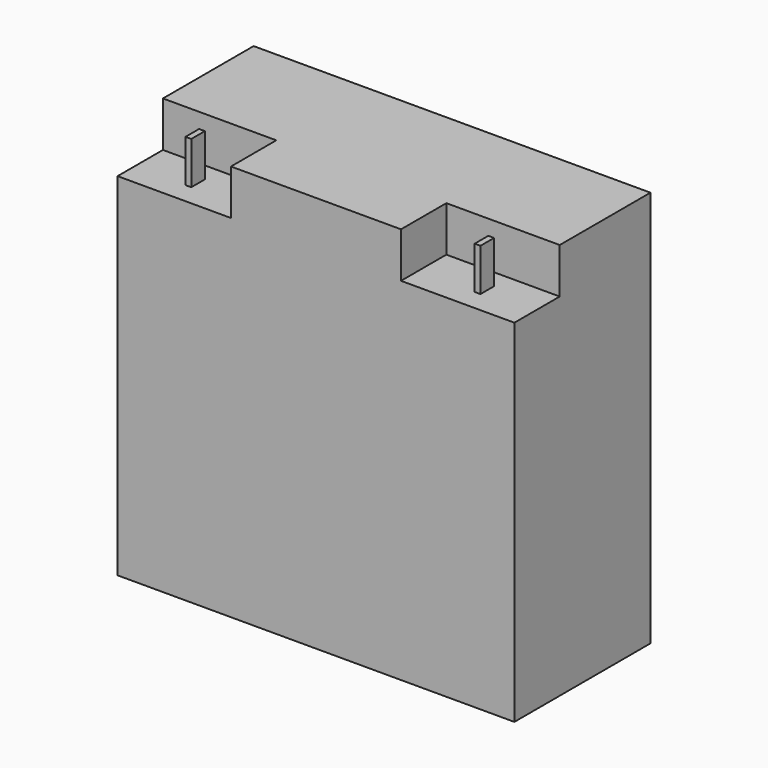
from build123d import *

# Parameters (mm, degrees)
F0_W     = 177.8
F0_H     = 76.2
F1_DEPTH = 177.8
F2_W     = 50.8
F2_H     = 25.4
F3_DEPTH = 20.32
F4_W     = 2.5917394697
F4_H     = 7.6049772211
F5_DEPTH = 19.05


# Not quite as in the source:
# - a length typed as a fraction of an inch, garbled in the dataset ("3 / 203.2 mm" for 3/8 in), is restored


with BuildPart() as f1:
    # F0 (on Top) → F1 (new body)
    with BuildSketch(Plane.XY):
        with Locations((-17.2624356211, 54.5294494442)):
            Rectangle(F0_W, F0_H)
    extrude(amount=F1_DEPTH)

    # F2 (on face) → F3 (cut)
    with BuildSketch(Plane.XY.offset(177.8)):
        with Locations((-80.7624356211, 29.1294494442)):
            Rectangle(F2_W, F2_H)
        with Locations((46.2375643789, 29.1294494442)):
            Rectangle(F2_W, F2_H)
    extrude(amount=-F3_DEPTH, mode=Mode.SUBTRACT)

    # F4 (on face) → F5 (join)
    with BuildSketch(Plane.XY.offset(157.48)):
        with Locations((-82.0583053559, 29.7569380547)):
            Rectangle(F4_W, F4_H)
    extrude(amount=F5_DEPTH)

    # F7: F1 across plane


with BuildPart() as f1_1:
    add(f1.part)
    add(f1.part.mirror(Plane(origin=(-17.2624356211, 55.5353900382, 85.7815841584), x_dir=(0, -1, 0), z_dir=(-1, 0, 0))))


solid = f1_1.part
